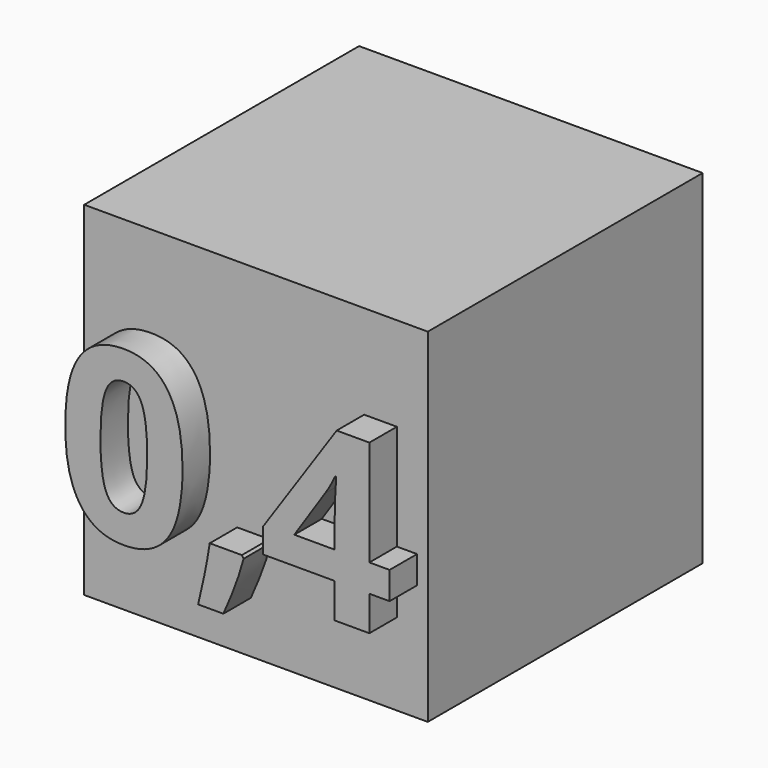
from build123d import *

# Parameters (mm, degrees)
F0_W         = 20
F0_H         = 20
F1_DEPTH     = 20
F2_TEXT_SIZE = 13.684875901
F3_DEPTH     = 2


# Not quite as in the source:
# - Text() gives the source's letters only with a copy of the font that has no kerning and outlines rounded to 1/6400 em; it was checked with that copy


with BuildPart() as f1:
    # F0 (on Front) → F1 (new body)
    with BuildSketch(Plane.XZ):
        with Locations((-10, 10)):
            Rectangle(F0_W, F0_H)
    extrude(amount=F1_DEPTH)

    # F2 (on face) → F3 (join)
    with BuildSketch(Plane.XZ.offset(20)):
        with Locations((-20, 4.7716200352)):
            Text('0,4', F2_TEXT_SIZE, font='Open Sans', font_style=FontStyle.BOLD, text_align=(TextAlign.LEFT, TextAlign.BOTTOM))
    extrude(amount=F3_DEPTH)


solid = f1.part
